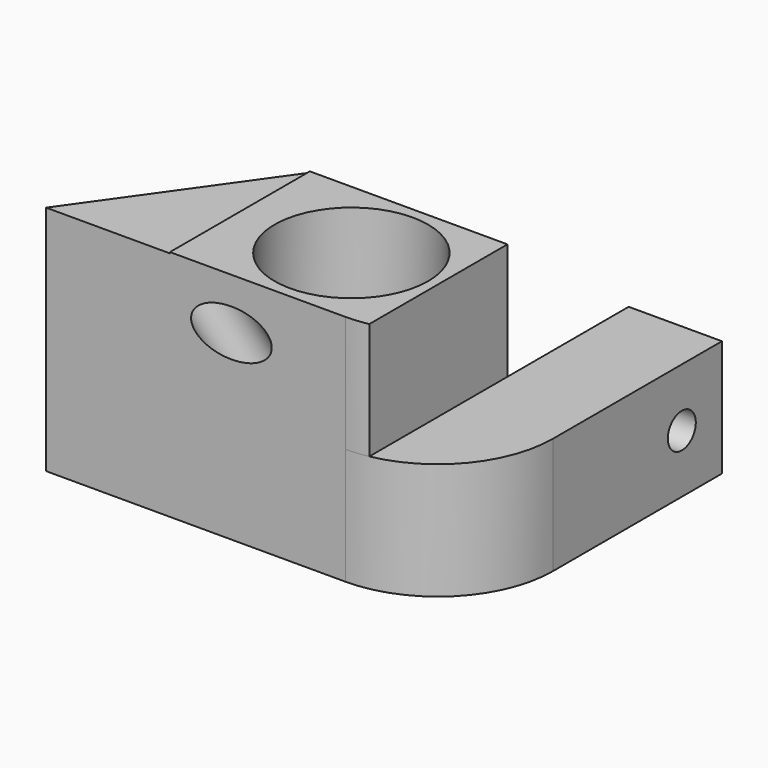
from build123d import *

# Parameters (mm, degrees)
F0_W     = 8
F0_H     = 13
F1_DEPTH = 10
F2_R     = 9.898276
F4_D     = 3
F5_R     = 6.582454
F6_DEPTH = 10
F7_DEPTH = 19.9
F9_D     = 4


with BuildPart() as f1:
    # F0 (on Top) → F1 (new body)
    with BuildSketch(Plane.XY):
        with Locations((-3.28516, 8.54833)):
            Rectangle(F0_W, F0_H)
        with BuildLine():
            Line((0.71484, 2.04833), (-7.28516, 2.04833))
            Line((-7.28516, 2.04833), (-24.237746, 2.04833))
            Line((-24.237746, 2.04833), (-24.237746, -5.45167))
            Line((-24.237746, -5.45167), (-21.257105, -5.45167))
            ThreePointArc((-21.257105, -5.45167), (-14.674651, 1.130784), (-8.092197, -5.45167))
            Line((-8.092197, -5.45167), (0.71484, -5.45167))
            Line((0.71484, -5.45167), (0.71484, 2.04833))
        make_face()
        with BuildLine():
            Line((0.71484, -12.95167), (0.71484, -5.45167))
            Line((0.71484, -5.45167), (-8.092197, -5.45167))
            ThreePointArc((-8.092197, -5.45167), (-14.674651, -12.034124), (-21.257105, -5.45167))
            Line((-21.257105, -5.45167), (-24.237746, -5.45167))
            Line((-24.237746, -5.45167), (-24.237746, -12.95167))
            Line((-24.237746, -12.95167), (0.71484, -12.95167))
        make_face()
    extrude(amount=F1_DEPTH)

    # F2
    f2_edges = [f1.edges().sort_by_distance(p)[0] for p in [
        (0.71484, -12.95167, 5),
    ]]
    fillet(f2_edges, radius=F2_R)

    # F4 (through all)
    with Locations(Plane(origin=(-7.28516, 0, 0), x_dir=(0, -1, 0), z_dir=(-1, 0, 0))):
        with Locations((-10.748397, 5)):
            Hole(F4_D / 2)

    # F5 (on face) → F6 (join)
    with BuildSketch(Plane.XY.offset(10)):
        with BuildLine():
            Line((-7.28516, -12.767941), (-7.28516, 2.04833))
            Line((-7.28516, 2.04833), (-24.237746, 2.04833))
            Line((-24.237746, 2.04833), (-24.237746, -12.95167))
            Line((-24.237746, -12.95167), (-9.183435, -12.95167))
            ThreePointArc((-9.183435, -12.95167), (-8.229862, -12.905631), (-7.28516, -12.767941))
        make_face()
        with Locations((-14.674651, -5.45167)):
            Circle(F5_R, mode=Mode.SUBTRACT)
    extrude(amount=F6_DEPTH)

    # F0 (on Top) → F7 (join)
    with BuildSketch(Plane.XY):
        Polygon((-24.237746, -5.45167), (-24.237746, 2.04833), (-34.864664, -12.95167), (-24.237746, -12.95167), align=None)
    extrude(amount=F7_DEPTH)

    # F9 (through all)
    with Locations(Plane(origin=(-17.104077, 12.117575, 0), x_dir=(-0.578087, -0.815975, 0), z_dir=(-0.815975, 0.578087, 0))):
        with Locations((21.53159, 15.607167)):
            Hole(F9_D / 2)


solid = f1.part
